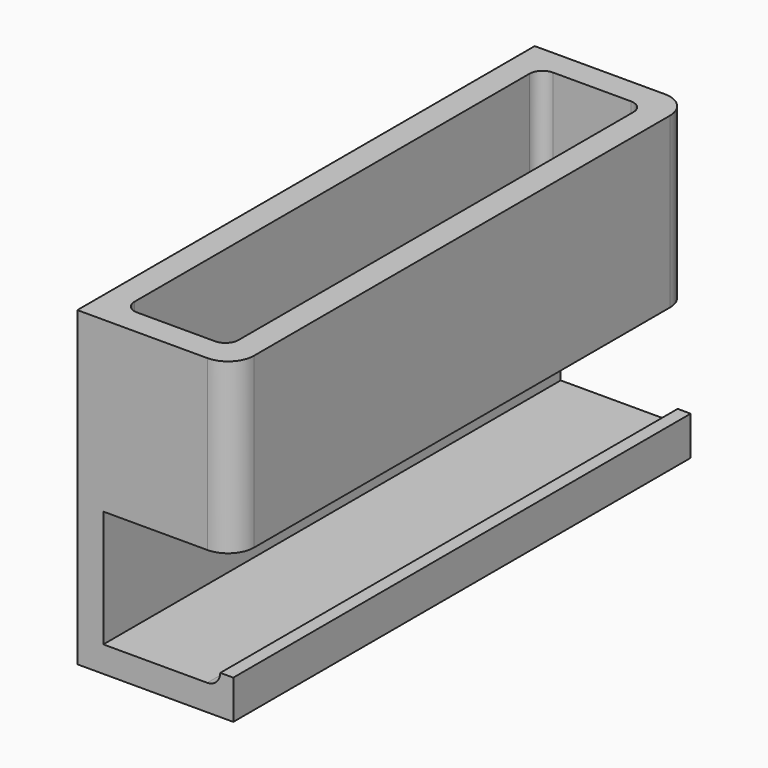
from build123d import *

# Parameters (mm, degrees)
F1_DEPTH = 110
F2_W     = 40
F2_H     = 200
F3_DEPTH = 60
F4_R     = 4.99999
F5_R     = 10


# Not quite as in the source:
# - a fillet or chamfer is up to 0.001 mm smaller than in the source, because OpenCascade refuses the exact size


with BuildPart() as f1:
    # F0 (on Front) → F1 (new body, symmetric)
    with BuildSketch(Plane.XZ):
        Polygon((-30, -60), (30, -60), (30, -50), (30, -45), (25, -45), (25, -50), (-20, -50), (-20, -5), (30, -5), (30, 60), (-30, 60), align=None)
    extrude(amount=F1_DEPTH, both=True)

    # F2 (on face) → F3 (cut)
    with BuildSketch(Plane.XY.offset(60)):
        Rectangle(F2_W, F2_H)
    extrude(amount=-F3_DEPTH, mode=Mode.SUBTRACT)

    # F4 (radius 5 in the source; OpenCascade refuses exactly that, so slightly less here)
    f4_edges = [f1.edges().sort_by_distance(p)[0] for p in [
        (-20, 100, 30),
        (20, 100, 30),
        (-20, -100, 30),
        (20, -100, 30),
        (25, 0, -50),
    ]]
    fillet(f4_edges, radius=F4_R)

    # F5
    f5_edges = [f1.edges().sort_by_distance(p)[0] for p in [
        (30, -110, 27.5),
        (30, 110, 27.5),
    ]]
    fillet(f5_edges, radius=F5_R)


solid = f1.part
